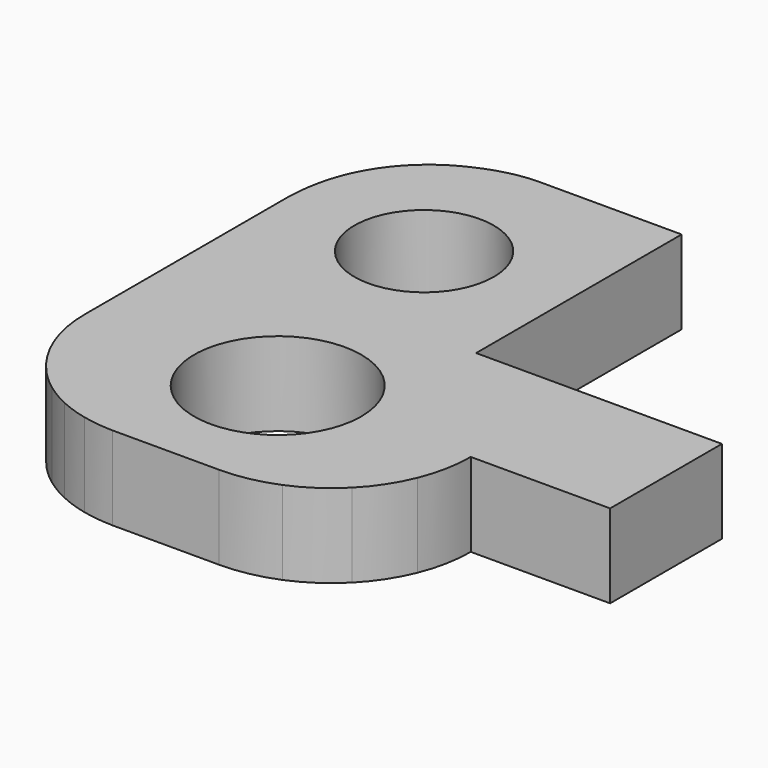
from build123d import *

# Parameters (mm, degrees)
F0_R     = 3
F0_R_2   = 2.5
F1_DEPTH = 3
F2_DEPTH = 5


# Not quite as in the source:
# - ends of sketch curves that miss each other by under 0.0002 mm in the source are joined


with BuildPart() as f1:
    # F0 (on Top) → F1 (new body)
    with BuildSketch(Plane.XY):
        with BuildLine():
            Line((-1.7219635134, -9.6237825349), (-1.7162322612, -9.6237825349))
            Line((-1.7162322612, -9.6237825349), (2.1097812593, -9.6237806245))
            ThreePointArc((2.1097812593, -9.6237806245), (3.109244006, -9.5259463757), (4.0703036603, -9.2346361811))
            ThreePointArc((4.0703036603, -9.2346361811), (4.9367767363, -8.7689594925), (5.6928675676, -8.1397082139))
            ThreePointArc((5.6928675676, -8.1397082139), (6.3014355553, -7.384861889), (6.7518423579, -6.5262108466))
            ThreePointArc((6.7518423579, -6.5262108466), (7.0313366054, -5.5856490766), (7.1251796223, -4.6089367858))
            Line((7.1251796223, -4.6089367858), (7.1251795967, 0.4059089633))
            Line((7.1251795967, 0.4059089633), (3.3043447402, 0.4059089633))
            Line((3.3043447402, 0.4059089633), (3.3043447402, 9.6236730545))
            Line((3.3043447402, 9.6236730545), (-1.7092449094, 9.6236835618))
            ThreePointArc((-1.7092449094, 9.6236835618), (-2.0928177445, 9.6100571875), (-2.4738865464, 9.5642275806))
            ThreePointArc((-2.4738865464, 9.5642275806), (-2.8609393666, 9.4846946207), (-3.2402037336, 9.3738166285))
            ThreePointArc((-3.2402037336, 9.3738166285), (-3.6975405848, 9.1984368029), (-4.1390265018, 8.9862923546))
            ThreePointArc((-4.1390265018, 8.9862923546), (-4.5162413892, 8.7629757089), (-4.8714990411, 8.5061617901))
            ThreePointArc((-4.8714990411, 8.5061617901), (-5.2720148148, 8.1490003263), (-5.6296128286, 7.7488742742))
            ThreePointArc((-5.6296128286, 7.7488742742), (-5.9394367718, 7.3112544614), (-6.197789407, 6.8414078072))
            ThreePointArc((-6.197789407, 6.8414078072), (-6.3173685837, 6.5707517714), (-6.4204719372, 6.2934007888))
            ThreePointArc((-6.4204719372, 6.2934007888), (-6.5129249786, 5.9920188156), (-6.5882375678, 5.6859033621))
            ThreePointArc((-6.5882375678, 5.6859033621), (-6.6481890942, 5.3652316519), (-6.6899638063, 5.0416896752))
            ThreePointArc((-6.6899638063, 5.0416896752), (-6.7168439977, 4.6824291061), (-6.7253469337, 4.3222646908))
            Line((-6.7253469337, 4.3222646908), (-6.7253324298, -4.6083307059))
            ThreePointArc((-6.7253324298, -4.6083307059), (-6.6405112105, -5.5189445936), (-6.3874853783, -6.3978019019))
            ThreePointArc((-6.3874853783, -6.3978019019), (-5.9650696712, -7.2398337428), (-5.3973270448, -7.9915790132))
            ThreePointArc((-5.3973270448, -7.9915790132), (-5.0455065065, -8.3419922854), (-4.6606937322, -8.6558175446))
            ThreePointArc((-4.6606937322, -8.6558175446), (-4.2509916029, -8.9267871137), (-3.8162055499, -9.1553509281))
            ThreePointArc((-3.8162055499, -9.1553509281), (-3.3266240966, -9.3511061983), (-2.8189514749, -9.4935092865))
            ThreePointArc((-2.8189514749, -9.4935092865), (-2.2737789347, -9.586614675), (-1.7219635134, -9.6237825349))
        make_face()
        with Locations((0.1967744991, -4.6086336082)):
            Circle(F0_R, mode=Mode.SUBTRACT)
        with Locations((-1.6951942668, 4.3222646911)):
            Circle(F0_R_2, mode=Mode.SUBTRACT)
    extrude(amount=-F1_DEPTH)

    # F2 (add): a face of the model
    f2_faces = [f1.faces().sort_by_distance(p)[0] for p in [
        (7.1251796095, -2.1015139113, -1.5),
    ]]
    extrude(f2_faces, amount=F2_DEPTH)


solid = f1.part
